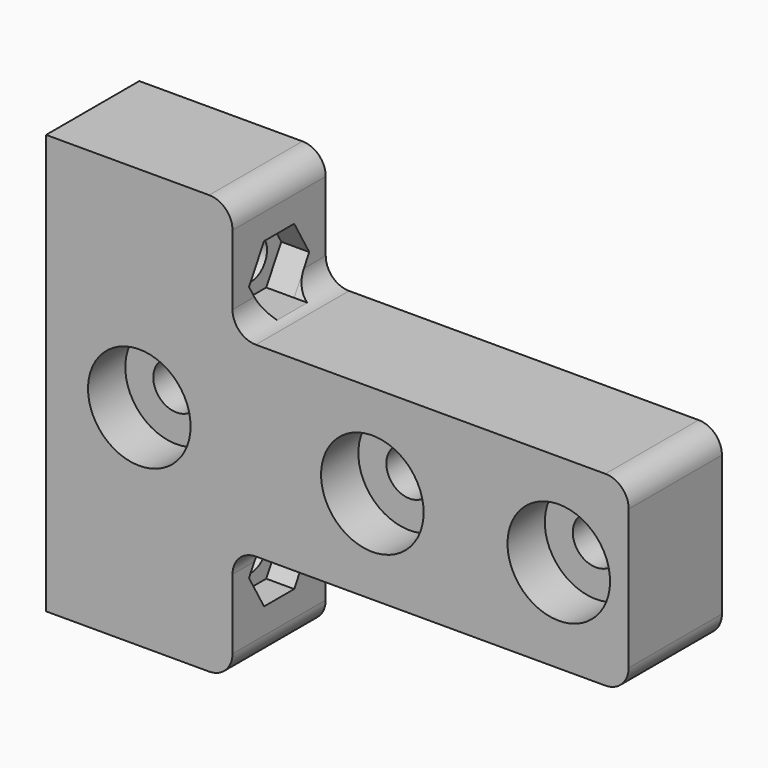
from build123d import *

# Parameters (mm, degrees)
F0_W          = 125
F0_H          = 40
F0_R          = 5
F1_DEPTH      = 25
F2_R          = 11
F3_DEPTH      = 10
F4_W          = 40
F4_H          = 25
F5_DEPTH      = 25
F6_R          = 4.25
F7_DEPTH      = 40
F9_DEPTH      = 6
F10_T4_DEPTH  = 25
F10_T10_DEPTH = 25
F10_T16_DEPTH = 25
F10_T23_DEPTH = 25
F10_T29_DEPTH = 25
F10_T35_DEPTH = 25
F10_T41_DEPTH = 25
F10_T47_DEPTH = 25
F10_T54_DEPTH = 25
F10_T60_DEPTH = 25
F10_T63_DEPTH = 50


# Not quite as in the source:
# - a fillet or chamfer that OpenCascade refuses, or shapes differently, is made with other operations: its cross-section is extruded or revolved along the edge and cut away or added


with BuildPart() as f1:
    # F0 (on Front) → F1 (new body)
    with BuildSketch(Plane.XZ):
        with Locations((-7.5, 0)):
            Rectangle(F0_W, F0_H)
        with Locations((-50, 0)):
            Circle(F0_R, mode=Mode.SUBTRACT)
        Circle(F0_R, mode=Mode.SUBTRACT)
        with Locations((40, 0)):
            Circle(F0_R, mode=Mode.SUBTRACT)
    extrude(amount=F1_DEPTH)

    # F2 (on face) → F3 (cut)
    with BuildSketch(Plane.XZ.offset(25)):
        with Locations((-50, 0)):
            Circle(F2_R)
        Circle(F2_R)
        with Locations((40, 0)):
            Circle(F2_R)
    extrude(amount=-F3_DEPTH, mode=Mode.SUBTRACT)

    # F4 (on face) → F5 (join)
    with BuildSketch(Plane(origin=(0, 0, 0), x_dir=(-1, 0, 0), z_dir=(0, 1, 0))):
        with Locations((50, 32.5)):
            Rectangle(F4_W, F4_H)
        with Locations((50, -32.5)):
            Rectangle(F4_W, F4_H)
    extrude(amount=-F5_DEPTH)

    # F6 (on face) → F7 (cut, through all)
    with BuildSketch(Plane(origin=(-70, 0, 0), x_dir=(0, -1, 0), z_dir=(-1, 0, 0))):
        with Locations((12.5, 27.5)):
            Circle(F6_R)
        with Locations((12.5, -27.5)):
            Circle(F6_R)
    extrude(amount=-F7_DEPTH, mode=Mode.SUBTRACT)

    # F8 (on face) → F9 (cut)
    with BuildSketch(Plane.YZ.offset(-30)):
        Polygon((-8.4585481157, 34.5), (-16.5414518843, 34.5), (-20.5829037687, 27.5), (-16.5414518843, 20.5), (-8.4585481157, 20.5), (-4.4170962313, 27.5), align=None)
        Polygon((-8.4585481157, -20.5), (-16.5414518843, -20.5), (-20.5829037687, -27.5), (-16.5414518843, -34.5), (-8.4585481157, -34.5), (-4.4170962313, -27.5), align=None)
    extrude(amount=-F9_DEPTH, mode=Mode.SUBTRACT)

    # F10: fillet of radius 5 on 6 edges, made by hand


with BuildPart() as f10_tool2:
    # F10_s3 → F10_t4 (new body)
    with BuildSketch(Plane.XZ):
        with BuildLine():
            ThreePointArc((-25, 20), (-28.5355339059, 21.4644660941), (-30, 25))
            Line((-30, 25), (-30, 20))
            Line((-30, 20), (-25, 20))
        make_face()
    extrude(amount=F10_T4_DEPTH)

    split(bisect_by=Plane.XY.offset(20.5), keep=Keep.BOTTOM)

    split(bisect_by=Plane(origin=(0, -15.2206714755, 8.7876587737), x_dir=(1, 0, 0), z_dir=(0, 0.8660254038, -0.5)), keep=Keep.TOP)


with BuildPart() as f1_1:
    add(f1.part)

    # F10_t1: union F10_tool2
    add(f10_tool2.part)


with BuildPart() as f10_tool8:
    # F10_s9 → F10_t10 (new body)
    with BuildSketch(Plane.XZ):
        with BuildLine():
            ThreePointArc((-25, 20), (-28.5355339059, 21.4644660941), (-30, 25))
            Line((-30, 25), (-30, 20))
            Line((-30, 20), (-25, 20))
        make_face()
    extrude(amount=F10_T10_DEPTH)

    split(bisect_by=Plane.XY.offset(20.5), keep=Keep.TOP)

    split(bisect_by=Plane(origin=(0, -15.2206714755, 8.7876587737), x_dir=(1, 0, 0), z_dir=(0, 0.8660254038, -0.5)), keep=Keep.TOP)


with BuildPart() as f1_2:
    add(f1_1.part)

    # F10_t7: union F10_tool8
    add(f10_tool8.part)


with BuildPart() as f10_tool14:
    # F10_s15 → F10_t16 (new body)
    with BuildSketch(Plane.XZ):
        with BuildLine():
            ThreePointArc((-25, 20), (-28.5355339059, 21.4644660941), (-30, 25))
            Line((-30, 25), (-30, 20))
            Line((-30, 20), (-25, 20))
        make_face()
    extrude(amount=F10_T16_DEPTH)

    split(bisect_by=Plane(origin=(0, -3.5293285245, -2.0376587737), x_dir=(1, 0, 0), z_dir=(0, 0.8660254038, 0.5)), keep=Keep.TOP)

    split(bisect_by=Plane.XY.offset(20.5), keep=Keep.BOTTOM)

    split(bisect_by=Plane(origin=(0, -15.2206714755, 8.7876587737), x_dir=(1, 0, 0), z_dir=(0, -0.8660254038, 0.5)), keep=Keep.TOP)


with BuildPart() as f1_3:
    add(f1_2.part)

    # F10_t13: union F10_tool14
    add(f10_tool14.part)


with BuildPart() as f10_tool21:
    # F10_s22 → F10_t23 (new body)
    with BuildSketch(Plane.XZ):
        with BuildLine():
            ThreePointArc((-25, 20), (-28.5355339059, 21.4644660941), (-30, 25))
            Line((-30, 25), (-30, 20))
            Line((-30, 20), (-25, 20))
        make_face()
    extrude(amount=F10_T23_DEPTH)

    split(bisect_by=Plane(origin=(0, -3.5293285245, -2.0376587737), x_dir=(1, 0, 0), z_dir=(0, -0.8660254038, -0.5)), keep=Keep.TOP)

    split(bisect_by=Plane.XY.offset(20.5), keep=Keep.BOTTOM)


with BuildPart() as f1_4:
    add(f1_3.part)

    # F10_t20: union F10_tool21
    add(f10_tool21.part)


with BuildPart() as f10_tool27:
    # F10_s28 → F10_t29 (new body)
    with BuildSketch(Plane.XZ):
        with BuildLine():
            ThreePointArc((-25, 20), (-28.5355339059, 21.4644660941), (-30, 25))
            Line((-30, 25), (-30, 20))
            Line((-30, 20), (-25, 20))
        make_face()
    extrude(amount=F10_T29_DEPTH)

    split(bisect_by=Plane(origin=(0, -3.5293285245, -2.0376587737), x_dir=(1, 0, 0), z_dir=(0, -0.8660254038, -0.5)), keep=Keep.TOP)

    split(bisect_by=Plane.XY.offset(20.5), keep=Keep.TOP)


with BuildPart() as f1_5:
    add(f1_4.part)

    # F10_t26: union F10_tool27
    add(f10_tool27.part)


with BuildPart() as f10_tool33:
    # F10_s34 → F10_t35 (new body)
    with BuildSketch(Plane.XZ):
        with BuildLine():
            ThreePointArc((-25, -20), (-28.5355339059, -21.4644660941), (-30, -25))
            Line((-30, -25), (-30, -20))
            Line((-30, -20), (-25, -20))
        make_face()
    extrude(amount=F10_T35_DEPTH)

    split(bisect_by=Plane.XY.offset(-20.5), keep=Keep.TOP)

    split(bisect_by=Plane(origin=(0, -15.2206714755, -8.7876587737), x_dir=(1, 0, 0), z_dir=(0, 0.8660254038, 0.5)), keep=Keep.TOP)


with BuildPart() as f1_6:
    add(f1_5.part)

    # F10_t32: union F10_tool33
    add(f10_tool33.part)


with BuildPart() as f10_tool39:
    # F10_s40 → F10_t41 (new body)
    with BuildSketch(Plane.XZ):
        with BuildLine():
            ThreePointArc((-25, -20), (-28.5355339059, -21.4644660941), (-30, -25))
            Line((-30, -25), (-30, -20))
            Line((-30, -20), (-25, -20))
        make_face()
    extrude(amount=F10_T41_DEPTH)

    split(bisect_by=Plane.XY.offset(-20.5), keep=Keep.BOTTOM)

    split(bisect_by=Plane(origin=(0, -15.2206714755, -8.7876587737), x_dir=(1, 0, 0), z_dir=(0, 0.8660254038, 0.5)), keep=Keep.TOP)


with BuildPart() as f1_7:
    add(f1_6.part)

    # F10_t38: union F10_tool39
    add(f10_tool39.part)


with BuildPart() as f10_tool45:
    # F10_s46 → F10_t47 (new body)
    with BuildSketch(Plane.XZ):
        with BuildLine():
            ThreePointArc((-25, -20), (-28.5355339059, -21.4644660941), (-30, -25))
            Line((-30, -25), (-30, -20))
            Line((-30, -20), (-25, -20))
        make_face()
    extrude(amount=F10_T47_DEPTH)

    split(bisect_by=Plane.XY.offset(-20.5), keep=Keep.TOP)

    split(bisect_by=Plane(origin=(0, -3.5293285245, 2.0376587737), x_dir=(1, 0, 0), z_dir=(0, 0.8660254038, -0.5)), keep=Keep.TOP)

    split(bisect_by=Plane(origin=(0, -15.2206714755, -8.7876587737), x_dir=(1, 0, 0), z_dir=(0, -0.8660254038, -0.5)), keep=Keep.TOP)


with BuildPart() as f1_8:
    add(f1_7.part)

    # F10_t44: union F10_tool45
    add(f10_tool45.part)


with BuildPart() as f10_tool52:
    # F10_s53 → F10_t54 (new body)
    with BuildSketch(Plane.XZ):
        with BuildLine():
            ThreePointArc((-25, -20), (-28.5355339059, -21.4644660941), (-30, -25))
            Line((-30, -25), (-30, -20))
            Line((-30, -20), (-25, -20))
        make_face()
    extrude(amount=F10_T54_DEPTH)

    split(bisect_by=Plane.XY.offset(-20.5), keep=Keep.TOP)

    split(bisect_by=Plane(origin=(0, -3.5293285245, 2.0376587737), x_dir=(1, 0, 0), z_dir=(0, -0.8660254038, 0.5)), keep=Keep.TOP)


with BuildPart() as f1_9:
    add(f1_8.part)

    # F10_t51: union F10_tool52
    add(f10_tool52.part)


with BuildPart() as f10_tool58:
    # F10_s59 → F10_t60 (new body)
    with BuildSketch(Plane.XZ):
        with BuildLine():
            ThreePointArc((-25, -20), (-28.5355339059, -21.4644660941), (-30, -25))
            Line((-30, -25), (-30, -20))
            Line((-30, -20), (-25, -20))
        make_face()
    extrude(amount=F10_T60_DEPTH)

    split(bisect_by=Plane.XY.offset(-20.5), keep=Keep.BOTTOM)

    split(bisect_by=Plane(origin=(0, -3.5293285245, 2.0376587737), x_dir=(1, 0, 0), z_dir=(0, -0.8660254038, 0.5)), keep=Keep.TOP)


with BuildPart() as f1_10:
    add(f1_9.part)

    # F10_t57: union F10_tool58
    add(f10_tool58.part)

    # F10_s64 → F10_t63 (cut)
    with BuildSketch(Plane.XZ.offset(-12.5)):
        with BuildLine():
            ThreePointArc((-35, 45), (-31.4644660941, 43.5355339059), (-30, 40))
            Line((-30, 40), (-30, 45))
            Line((-30, 45), (-35, 45))
        make_face()
        with BuildLine():
            ThreePointArc((-30, -40), (-31.4644660941, -43.5355339059), (-35, -45))
            Line((-35, -45), (-30, -45))
            Line((-30, -45), (-30, -40))
        make_face()
        with BuildLine():
            ThreePointArc((55, -15), (53.5355339059, -18.5355339059), (50, -20))
            Line((50, -20), (55, -20))
            Line((55, -20), (55, -15))
        make_face()
        with BuildLine():
            ThreePointArc((55, 15), (53.5355339059, 18.5355339059), (50, 20))
            Line((50, 20), (55, 20))
            Line((55, 20), (55, 15))
        make_face()
    extrude(amount=F10_T63_DEPTH, mode=Mode.SUBTRACT)


solid = f1_10.part
